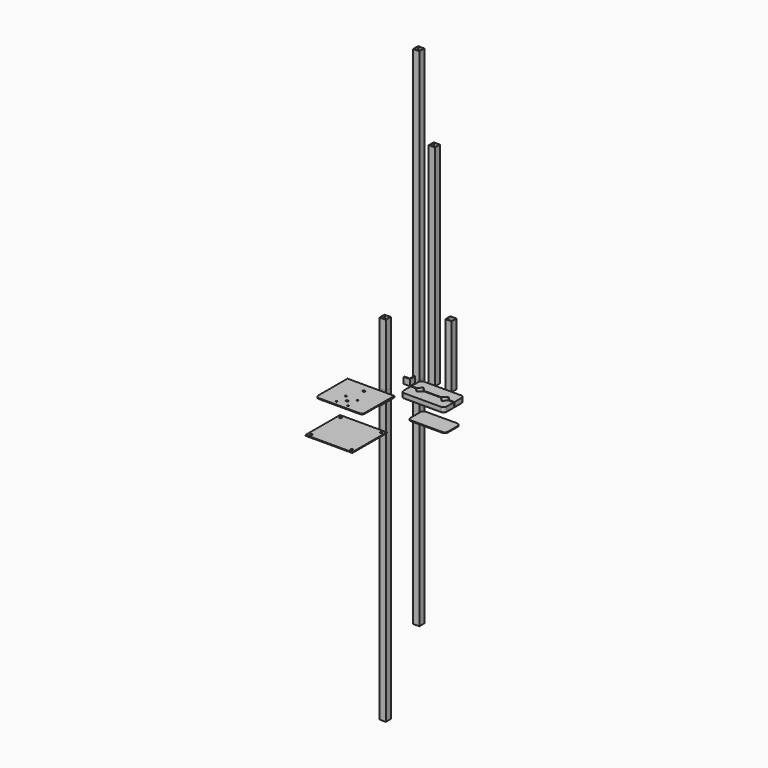
from build123d import *

# Parameters (mm, degrees)
F0_W      = 25.4
F0_H      = 25.4
F1_DEPTH  = 1181.1
F2_DEPTH  = 856.615
F3_DEPTH  = 25.4
F0_R      = 4.7625
F4_DEPTH  = 15.875
F5_DEPTH  = 3.175
F8_DEPTH  = 254
F10_DEPTH = 254
F11_DEPTH = 1187.45
F12_DEPTH = 880.2878
F0_R_2    = 3.175
F13_DEPTH = 3.175
F14_DEPTH = 3.175
F0_W_2    = 190.5
F0_H_2    = 175.514
F15_DEPTH = 3.175
F16_DEPTH = 3.175


# Not quite as in the source:
# - a feature names something its author has since deleted; it is built from what else it names


with BuildPart() as f1:
    # F0 (on Top) → F1 (new body)
    with BuildSketch(Plane.XY):
        with Locations((-44.022594732, 33.2031734467)):
            Rectangle(F0_W, F0_H)
        with BuildLine():
            ThreePointArc((-55.135094732, 42.7281734467), (-54.6701267472, 43.8507054618), (-53.547594732, 44.3156734467))
            Line((-53.547594732, 44.3156734467), (-34.497594732, 44.3156734467))
            ThreePointArc((-34.497594732, 44.3156734467), (-33.3750627169, 43.8507054618), (-32.910094732, 42.7281734467))
            Line((-32.910094732, 42.7281734467), (-32.910094732, 23.6781734467))
            ThreePointArc((-32.910094732, 23.6781734467), (-33.3750627169, 22.5556414315), (-34.497594732, 22.0906734467))
            Line((-34.497594732, 22.0906734467), (-53.547594732, 22.0906734467))
            ThreePointArc((-53.547594732, 22.0906734467), (-54.6701267472, 22.5556414315), (-55.135094732, 23.6781734467))
            Line((-55.135094732, 23.6781734467), (-55.135094732, 42.7281734467))
        make_face(mode=Mode.SUBTRACT)
    extrude(amount=F1_DEPTH)


with BuildPart() as f2:
    # F0 (on Top) → F2 (new body)
    with BuildSketch(Plane.XY):
        with Locations((19.2820195436, 33.6916345775)):
            Rectangle(F0_W, F0_H)
        with BuildLine():
            ThreePointArc((28.8070195436, 44.8041345775), (29.9295515588, 44.3391665926), (30.3945195436, 43.2166345775))
            Line((30.3945195436, 43.2166345775), (30.3945195436, 24.1666345775))
            ThreePointArc((30.3945195436, 24.1666345775), (29.9295515588, 23.0441025624), (28.8070195436, 22.5791345775))
            Line((28.8070195436, 22.5791345775), (9.7570195436, 22.5791345775))
            ThreePointArc((9.7570195436, 22.5791345775), (8.6344875285, 23.0441025624), (8.1695195436, 24.1666345775))
            Line((8.1695195436, 24.1666345775), (8.1695195436, 43.2166345775))
            ThreePointArc((8.1695195436, 43.2166345775), (8.6344875285, 44.3391665926), (9.7570195436, 44.8041345775))
            Line((9.7570195436, 44.8041345775), (28.8070195436, 44.8041345775))
        make_face(mode=Mode.SUBTRACT)
    extrude(amount=F2_DEPTH)


with BuildPart() as f3:
    # F0 (on Top) → F3 (new body)
    with BuildSketch(Plane.XY):
        with BuildLine():
            Line((-30.7852902532, -2.1858640671), (-33.9602902532, -2.1858640671))
            Line((-33.9602902532, -2.1858640671), (-33.9602902532, -21.2358640671))
            ThreePointArc((-33.9602902532, -21.2358640671), (-34.8902262229, -23.4809280973), (-37.1352902532, -24.4108640671))
            Line((-37.1352902532, -24.4108640671), (-56.1852902532, -24.4108640671))
            Line((-56.1852902532, -24.4108640671), (-56.1852902532, -27.5858640671))
            Line((-56.1852902532, -27.5858640671), (-30.7852902532, -27.5858640671))
            Line((-30.7852902532, -27.5858640671), (-30.7852902532, -2.1858640671))
        make_face()
    extrude(amount=F3_DEPTH)


with BuildPart() as f4:
    # F0 (on Top) → F4 (new body)
    with BuildSketch(Plane.XY):
        with BuildLine():
            Line((153.8100352997, 1.1835222483), (3.6851863311, 1.1835222483))
            ThreePointArc((3.6851863311, 1.1835222483), (-5.2950697899, -2.5362216307), (-9.0148136689, -11.5164777517))
            Line((-9.0148136689, -11.5164777517), (-9.0148136689, -48.0289777517))
            Line((-9.0148136689, -48.0289777517), (11.3940863311, -48.0289777517))
            Line((11.3940863311, -48.0289777517), (27.7670985733, -31.6559655096))
            Line((27.7670985733, -31.6559655096), (44.1401108154, -48.0289777517))
            Line((44.1401108154, -48.0289777517), (113.3551108154, -48.0289777517))
            Line((113.3551108154, -48.0289777517), (129.7281230576, -31.6559655096))
            Line((129.7281230576, -31.6559655096), (146.1011352997, -48.0289777517))
            Line((146.1011352997, -48.0289777517), (166.5100352997, -48.0289777517))
            Line((166.5100352997, -48.0289777517), (166.5100352997, -11.5164777517))
            ThreePointArc((166.5100352997, -11.5164777517), (162.7902914208, -2.5362216307), (153.8100352997, 1.1835222483))
        make_face()
        with Locations((3.6851863311, -11.5164777517)):
            Circle(F0_R, mode=Mode.SUBTRACT)
        with Locations((153.8100352997, -11.5164777517)):
            Circle(F0_R, mode=Mode.SUBTRACT)
        with Locations((3.6851863311, -11.5164777517)):
            Circle(F0_R)
        with Locations((153.8100352997, -11.5164777517)):
            Circle(F0_R)
    extrude(amount=F4_DEPTH)


with BuildPart() as f4b:
    # F0 (on Top) → F4, piece 2 (new body)
    with BuildSketch(Plane.XY):
        with BuildLine():
            Line((11.3940863311, -51.2039777517), (-9.0148136689, -51.2039777517))
            Line((-9.0148136689, -51.2039777517), (-9.0148136689, -87.7164777517))
            ThreePointArc((-9.0148136689, -87.7164777517), (-5.2950697899, -96.6967338728), (3.6851863311, -100.4164777517))
            Line((3.6851863311, -100.4164777517), (153.8100352997, -100.4164777517))
            ThreePointArc((153.8100352997, -100.4164777517), (162.7902914208, -96.6967338728), (166.5100352997, -87.7164777517))
            Line((166.5100352997, -87.7164777517), (166.5100352997, -51.2039777517))
            Line((166.5100352997, -51.2039777517), (146.1011352997, -51.2039777517))
            Line((146.1011352997, -51.2039777517), (129.7281230576, -67.5769899939))
            Line((129.7281230576, -67.5769899939), (113.3551108154, -51.2039777517))
            Line((113.3551108154, -51.2039777517), (44.1401108154, -51.2039777517))
            Line((44.1401108154, -51.2039777517), (27.7670985733, -67.5769899939))
            Line((27.7670985733, -67.5769899939), (11.3940863311, -51.2039777517))
        make_face()
        with Locations((3.6851863311, -87.7164777517)):
            Circle(F0_R, mode=Mode.SUBTRACT)
        with Locations((153.8100352997, -87.7164777517)):
            Circle(F0_R, mode=Mode.SUBTRACT)
        with Locations((153.8100352997, -87.7164777517)):
            Circle(F0_R)
        with Locations((3.6851863311, -87.7164777517)):
            Circle(F0_R)
    extrude(amount=F4_DEPTH)


with BuildPart() as f5:
    # F0 (on Top) → F5 (new body)
    with BuildSketch(Plane.XY):
        with BuildLine():
            Line((153.8100352997, 1.1835222483), (3.6851863311, 1.1835222483))
            ThreePointArc((3.6851863311, 1.1835222483), (-5.2950697899, -2.5362216307), (-9.0148136689, -11.5164777517))
            Line((-9.0148136689, -11.5164777517), (-9.0148136689, -48.0289777517))
            Line((-9.0148136689, -48.0289777517), (11.3940863311, -48.0289777517))
            Line((11.3940863311, -48.0289777517), (27.7670985733, -31.6559655096))
            Line((27.7670985733, -31.6559655096), (44.1401108154, -48.0289777517))
            Line((44.1401108154, -48.0289777517), (113.3551108154, -48.0289777517))
            Line((113.3551108154, -48.0289777517), (129.7281230576, -31.6559655096))
            Line((129.7281230576, -31.6559655096), (146.1011352997, -48.0289777517))
            Line((146.1011352997, -48.0289777517), (166.5100352997, -48.0289777517))
            Line((166.5100352997, -48.0289777517), (166.5100352997, -11.5164777517))
            ThreePointArc((166.5100352997, -11.5164777517), (162.7902914208, -2.5362216307), (153.8100352997, 1.1835222483))
        make_face()
        with Locations((3.6851863311, -11.5164777517)):
            Circle(F0_R, mode=Mode.SUBTRACT)
        with Locations((153.8100352997, -11.5164777517)):
            Circle(F0_R, mode=Mode.SUBTRACT)
        with BuildLine():
            Line((11.3940863311, -51.2039777517), (-9.0148136689, -51.2039777517))
            Line((-9.0148136689, -51.2039777517), (-9.0148136689, -87.7164777517))
            ThreePointArc((-9.0148136689, -87.7164777517), (-5.2950697899, -96.6967338728), (3.6851863311, -100.4164777517))
            Line((3.6851863311, -100.4164777517), (153.8100352997, -100.4164777517))
            ThreePointArc((153.8100352997, -100.4164777517), (162.7902914208, -96.6967338728), (166.5100352997, -87.7164777517))
            Line((166.5100352997, -87.7164777517), (166.5100352997, -51.2039777517))
            Line((166.5100352997, -51.2039777517), (146.1011352997, -51.2039777517))
            Line((146.1011352997, -51.2039777517), (129.7281230576, -67.5769899939))
            Line((129.7281230576, -67.5769899939), (113.3551108154, -51.2039777517))
            Line((113.3551108154, -51.2039777517), (44.1401108154, -51.2039777517))
            Line((44.1401108154, -51.2039777517), (27.7670985733, -67.5769899939))
            Line((27.7670985733, -67.5769899939), (11.3940863311, -51.2039777517))
        make_face()
        with Locations((3.6851863311, -87.7164777517)):
            Circle(F0_R, mode=Mode.SUBTRACT)
        with Locations((153.8100352997, -87.7164777517)):
            Circle(F0_R, mode=Mode.SUBTRACT)
        Polygon((113.3551108154, -48.0289777517), (44.1401108154, -48.0289777517), (45.7276108154, -49.6164777517), (44.1401108154, -51.2039777517), (113.3551108154, -51.2039777517), (111.7676108154, -49.6164777517), align=None)
        Polygon((11.3940863311, -48.0289777517), (-9.0148136689, -48.0289777517), (-9.0148136689, -51.2039777517), (11.3940863311, -51.2039777517), (9.8065863311, -49.6164777517), align=None)
        Polygon((166.5100352997, -51.2039777517), (166.5100352997, -48.0289777517), (146.1011352997, -48.0289777517), (147.6886352997, -49.6164777517), (146.1011352997, -51.2039777517), align=None)
        Polygon((27.7670985733, -31.6559655096), (11.3940863311, -48.0289777517), (44.1401108154, -48.0289777517), align=None)
        Polygon((44.1401108154, -48.0289777517), (11.3940863311, -48.0289777517), (9.8065863311, -49.6164777517), (11.3940863311, -51.2039777517), (44.1401108154, -51.2039777517), (45.7276108154, -49.6164777517), align=None)
        Polygon((44.1401108154, -51.2039777517), (11.3940863311, -51.2039777517), (27.7670985733, -67.5769899939), align=None)
        Polygon((129.7281230576, -67.5769899939), (146.1011352997, -51.2039777517), (113.3551108154, -51.2039777517), align=None)
        Polygon((147.6886352997, -49.6164777517), (146.1011352997, -48.0289777517), (113.3551108154, -48.0289777517), (111.7676108154, -49.6164777517), (113.3551108154, -51.2039777517), (146.1011352997, -51.2039777517), align=None)
        Polygon((113.3551108154, -48.0289777517), (146.1011352997, -48.0289777517), (129.7281230576, -31.6559655096), align=None)
    extrude(amount=-F5_DEPTH)


with BuildPart() as f8:
    # F0 (on Top) → F8 (new body)
    with BuildSketch(Plane.XY):
        with Locations((85.7311247587, 35.6169353843)):
            Rectangle(F0_W, F0_H)
        with BuildLine():
            Line((95.2561247587, 24.5044353843), (76.2061247587, 24.5044353843))
            ThreePointArc((76.2061247587, 24.5044353843), (75.0835927436, 24.9694033691), (74.6186247587, 26.0919353843))
            Line((74.6186247587, 26.0919353843), (74.6186247587, 45.1419353843))
            ThreePointArc((74.6186247587, 45.1419353843), (75.0835927436, 46.2644673994), (76.2061247587, 46.7294353843))
            Line((76.2061247587, 46.7294353843), (95.2561247587, 46.7294353843))
            ThreePointArc((95.2561247587, 46.7294353843), (96.3786567739, 46.2644673994), (96.8436247587, 45.1419353843))
            Line((96.8436247587, 45.1419353843), (96.8436247587, 26.0919353843))
            ThreePointArc((96.8436247587, 26.0919353843), (96.3786567739, 24.9694033691), (95.2561247587, 24.5044353843))
        make_face(mode=Mode.SUBTRACT)
    extrude(amount=F8_DEPTH)


with BuildPart() as f10:
    # F0 (on Top) → F10 (new body)
    with BuildSketch(Plane.XY):
        with Locations((-84.5126371503, -86.7445782954)):
            Rectangle(F0_W, F0_H)
        with BuildLine():
            ThreePointArc((-74.9876371503, -75.6320782954), (-73.8651051352, -76.0970462802), (-73.4001371503, -77.2195782954))
            Line((-73.4001371503, -77.2195782954), (-73.4001371503, -96.2695782954))
            ThreePointArc((-73.4001371503, -96.2695782954), (-73.8651051352, -97.3921103105), (-74.9876371503, -97.8570782954))
            Line((-74.9876371503, -97.8570782954), (-94.0376371503, -97.8570782954))
            ThreePointArc((-94.0376371503, -97.8570782954), (-95.1601691654, -97.3921103105), (-95.6251371503, -96.2695782954))
            Line((-95.6251371503, -96.2695782954), (-95.6251371503, -77.2195782954))
            ThreePointArc((-95.6251371503, -77.2195782954), (-95.1601691654, -76.0970462802), (-94.0376371503, -75.6320782954))
            Line((-94.0376371503, -75.6320782954), (-74.9876371503, -75.6320782954))
        make_face(mode=Mode.SUBTRACT)
    extrude(amount=F10_DEPTH)


with BuildPart() as f11:
    # F0 (on Top) → F11 (new body)
    with BuildSketch(Plane.XY):
        with Locations((-84.5126371503, -86.7445782954)):
            Rectangle(F0_W, F0_H)
        with BuildLine():
            ThreePointArc((-74.9876371503, -75.6320782954), (-73.8651051352, -76.0970462802), (-73.4001371503, -77.2195782954))
            Line((-73.4001371503, -77.2195782954), (-73.4001371503, -96.2695782954))
            ThreePointArc((-73.4001371503, -96.2695782954), (-73.8651051352, -97.3921103105), (-74.9876371503, -97.8570782954))
            Line((-74.9876371503, -97.8570782954), (-94.0376371503, -97.8570782954))
            ThreePointArc((-94.0376371503, -97.8570782954), (-95.1601691654, -97.3921103105), (-95.6251371503, -96.2695782954))
            Line((-95.6251371503, -96.2695782954), (-95.6251371503, -77.2195782954))
            ThreePointArc((-95.6251371503, -77.2195782954), (-95.1601691654, -76.0970462802), (-94.0376371503, -75.6320782954))
            Line((-94.0376371503, -75.6320782954), (-74.9876371503, -75.6320782954))
        make_face(mode=Mode.SUBTRACT)
    extrude(amount=-F11_DEPTH)


with BuildPart() as f12:
    # F0 (on Top) → F12 (new body)
    with BuildSketch(Plane.XY):
        with Locations((-44.022594732, 33.2031734467)):
            Rectangle(F0_W, F0_H)
        with BuildLine():
            ThreePointArc((-55.135094732, 42.7281734467), (-54.6701267472, 43.8507054618), (-53.547594732, 44.3156734467))
            Line((-53.547594732, 44.3156734467), (-34.497594732, 44.3156734467))
            ThreePointArc((-34.497594732, 44.3156734467), (-33.3750627169, 43.8507054618), (-32.910094732, 42.7281734467))
            Line((-32.910094732, 42.7281734467), (-32.910094732, 23.6781734467))
            ThreePointArc((-32.910094732, 23.6781734467), (-33.3750627169, 22.5556414315), (-34.497594732, 22.0906734467))
            Line((-34.497594732, 22.0906734467), (-53.547594732, 22.0906734467))
            ThreePointArc((-53.547594732, 22.0906734467), (-54.6701267472, 22.5556414315), (-55.135094732, 23.6781734467))
            Line((-55.135094732, 23.6781734467), (-55.135094732, 42.7281734467))
        make_face(mode=Mode.SUBTRACT)
    extrude(amount=-F12_DEPTH)


with BuildPart() as f13:
    # F0 (on Top) → F13 (new body)
    with BuildSketch(Plane.XY):
        with BuildLine():
            Line((-140.5062990204, -185.1695782954), (-215.0408358783, -185.1695782954))
            Line((-215.0408358783, -185.1695782954), (-215.0408358783, -264.5445782954))
            ThreePointArc((-215.0408358783, -264.5445782954), (-211.3210919994, -273.5248344164), (-202.3408358783, -277.2445782954))
            Line((-202.3408358783, -277.2445782954), (-37.2408358783, -277.2445782954))
            ThreePointArc((-37.2408358783, -277.2445782954), (-28.2605797572, -273.5248344164), (-24.5408358783, -264.5445782954))
            Line((-24.5408358783, -264.5445782954), (-24.5408358783, -185.1695782954))
            Line((-24.5408358783, -185.1695782954), (-100.3453727362, -185.1695782954))
            ThreePointArc((-100.3453727362, -185.1695782954), (-89.4333706631, -197.6441831176), (-85.5008358783, -213.7445782954))
            ThreePointArc((-85.5008358783, -213.7445782954), (-136.5262310561, -244.7370435106), (-140.5062990204, -185.1695782954))
        make_face()
        with Locations((-143.9990081961, -259.5427506132)):
            Circle(F0_R_2, mode=Mode.SUBTRACT)
        with Locations((-96.8526635605, -259.5427506132)):
            Circle(F0_R_2, mode=Mode.SUBTRACT)
        with Locations((-202.3408358783, -199.4570782954)):
            Circle(F0_R_2, mode=Mode.SUBTRACT)
        with Locations((-37.2408358783, -199.4570782954)):
            Circle(F0_R_2, mode=Mode.SUBTRACT)
        with BuildLine():
            Line((-37.2408358783, -115.3195782954), (-202.3408358783, -115.3195782954))
            Line((-202.3408358783, -115.3195782954), (-215.0408358783, -115.3195782954))
            Line((-215.0408358783, -115.3195782954), (-215.0408358783, -124.8445782954))
            Line((-215.0408358783, -124.8445782954), (-215.0408358783, -185.1695782954))
            Line((-215.0408358783, -185.1695782954), (-140.5062990204, -185.1695782954))
            ThreePointArc((-140.5062990204, -185.1695782954), (-120.4258358783, -178.8195782954), (-100.3453727362, -185.1695782954))
            Line((-100.3453727362, -185.1695782954), (-24.5408358783, -185.1695782954))
            Line((-24.5408358783, -185.1695782954), (-24.5408358783, -124.8445782954))
            Line((-24.5408358783, -124.8445782954), (-24.5408358783, -115.3195782954))
            Line((-24.5408358783, -115.3195782954), (-37.2408358783, -115.3195782954))
        make_face()
        with Locations((-202.3408358783, -145.4820782954)):
            Circle(F0_R_2, mode=Mode.SUBTRACT)
        Polygon((-171.4063481204, -168.2050905375), (-189.3668603626, -150.2445782954), (-171.4063481204, -132.2840660532), (-153.4458358783, -150.2445782954), align=None, mode=Mode.SUBTRACT)
        with Locations((-120.4258358783, -150.2445782954)):
            Circle(F0_R, mode=Mode.SUBTRACT)
        Polygon((-69.4453236362, -168.2050905375), (-87.4058358783, -150.2445782954), (-69.4453236362, -132.2840660532), (-51.484811394, -150.2445782954), align=None, mode=Mode.SUBTRACT)
        with Locations((-37.2408358783, -145.4820782954)):
            Circle(F0_R_2, mode=Mode.SUBTRACT)
        with BuildLine():
            Line((-100.3453727362, -185.1695782954), (-140.5062990204, -185.1695782954))
            ThreePointArc((-140.5062990204, -185.1695782954), (-136.5262310561, -244.7370435106), (-85.5008358783, -213.7445782954))
            ThreePointArc((-85.5008358783, -213.7445782954), (-89.4333706631, -197.6441831176), (-100.3453727362, -185.1695782954))
        make_face()
        with Locations((-120.4258358783, -235.9695782954)):
            Circle(F0_R, mode=Mode.SUBTRACT)
        with Locations((-143.9990081961, -212.3964059776)):
            Circle(F0_R_2, mode=Mode.SUBTRACT)
        with Locations((-96.8526635605, -212.3964059776)):
            Circle(F0_R_2, mode=Mode.SUBTRACT)
        Polygon((-171.4063481204, -132.2840660532), (-189.3668603626, -150.2445782954), (-171.4063481204, -168.2050905375), (-153.4458358783, -150.2445782954), align=None)
        Polygon((-69.4453236362, -132.2840660532), (-87.4058358783, -150.2445782954), (-69.4453236362, -168.2050905375), (-51.484811394, -150.2445782954), align=None)
        with BuildLine():
            ThreePointArc((-100.3453727362, -185.1695782954), (-120.4258358783, -178.8195782954), (-140.5062990204, -185.1695782954))
            Line((-140.5062990204, -185.1695782954), (-100.3453727362, -185.1695782954))
        make_face()
        with Locations((-202.3408358783, -145.4820782954)):
            Circle(F0_R_2)
        with Locations((-202.3408358783, -199.4570782954)):
            Circle(F0_R_2)
        with Locations((-37.2408358783, -199.4570782954)):
            Circle(F0_R_2)
        with Locations((-37.2408358783, -145.4820782954)):
            Circle(F0_R_2)
    extrude(amount=F13_DEPTH)


with BuildPart() as f14:
    # F0 (on Top) → F14 (new body)
    with BuildSketch(Plane.XY):
        with BuildLine():
            Line((-37.2408358783, -115.3195782954), (-202.3408358783, -115.3195782954))
            Line((-202.3408358783, -115.3195782954), (-215.0408358783, -115.3195782954))
            Line((-215.0408358783, -115.3195782954), (-215.0408358783, -124.8445782954))
            Line((-215.0408358783, -124.8445782954), (-215.0408358783, -185.1695782954))
            Line((-215.0408358783, -185.1695782954), (-140.5062990204, -185.1695782954))
            ThreePointArc((-140.5062990204, -185.1695782954), (-120.4258358783, -178.8195782954), (-100.3453727362, -185.1695782954))
            Line((-100.3453727362, -185.1695782954), (-24.5408358783, -185.1695782954))
            Line((-24.5408358783, -185.1695782954), (-24.5408358783, -124.8445782954))
            Line((-24.5408358783, -124.8445782954), (-24.5408358783, -115.3195782954))
            Line((-24.5408358783, -115.3195782954), (-37.2408358783, -115.3195782954))
        make_face()
        with Locations((-202.3408358783, -145.4820782954)):
            Circle(F0_R_2, mode=Mode.SUBTRACT)
        Polygon((-171.4063481204, -168.2050905375), (-189.3668603626, -150.2445782954), (-171.4063481204, -132.2840660532), (-153.4458358783, -150.2445782954), align=None, mode=Mode.SUBTRACT)
        with Locations((-120.4258358783, -150.2445782954)):
            Circle(F0_R, mode=Mode.SUBTRACT)
        Polygon((-69.4453236362, -168.2050905375), (-87.4058358783, -150.2445782954), (-69.4453236362, -132.2840660532), (-51.484811394, -150.2445782954), align=None, mode=Mode.SUBTRACT)
        with Locations((-37.2408358783, -145.4820782954)):
            Circle(F0_R_2, mode=Mode.SUBTRACT)
        Polygon((-171.4063481204, -132.2840660532), (-189.3668603626, -150.2445782954), (-171.4063481204, -168.2050905375), (-153.4458358783, -150.2445782954), align=None)
        Polygon((-69.4453236362, -132.2840660532), (-87.4058358783, -150.2445782954), (-69.4453236362, -168.2050905375), (-51.484811394, -150.2445782954), align=None)
        with Locations((-202.3408358783, -145.4820782954)):
            Circle(F0_R_2)
        with Locations((-37.2408358783, -145.4820782954)):
            Circle(F0_R_2)
    extrude(amount=-F14_DEPTH)


with BuildPart() as f15:
    # F0 (on Top) → F15 (new body)
    with BuildSketch(Plane.XY):
        with Locations((18.171196328, -413.6125734582)):
            Rectangle(F0_W_2, F0_H_2)
        with Locations((-64.378803672, -488.6695734582)):
            Circle(F0_R, mode=Mode.SUBTRACT)
        with Locations((-64.378803672, -338.5555734582)):
            Circle(F0_R, mode=Mode.SUBTRACT)
        with Locations((100.721196328, -488.6695734582)):
            Circle(F0_R, mode=Mode.SUBTRACT)
        with Locations((100.721196328, -338.5555734582)):
            Circle(F0_R, mode=Mode.SUBTRACT)
    extrude(amount=F15_DEPTH)


with BuildPart() as f16:
    # F0 (on Top) → F16 (new body)
    with BuildSketch(Plane.XY):
        with BuildLine():
            Line((249.7534018952, -137.7315354975), (122.7534018952, -137.7315354975))
            ThreePointArc((122.7534018952, -137.7315354975), (113.7731457742, -141.4512793764), (110.0534018952, -150.4315354975))
            Line((110.0534018952, -150.4315354975), (110.0534018952, -201.2315354975))
            ThreePointArc((110.0534018952, -201.2315354975), (113.7731457742, -210.2117916186), (122.7534018952, -213.9315354975))
            Line((122.7534018952, -213.9315354975), (249.7534018952, -213.9315354975))
            ThreePointArc((249.7534018952, -213.9315354975), (258.7336580163, -210.2117916186), (262.4534018952, -201.2315354975))
            Line((262.4534018952, -201.2315354975), (262.4534018952, -150.4315354975))
            ThreePointArc((262.4534018952, -150.4315354975), (258.7336580163, -141.4512793764), (249.7534018952, -137.7315354975))
        make_face()
        Polygon((135.2728896531, -193.7920477396), (117.312377411, -175.8315354975), (135.2728896531, -157.8710232554), (153.2334018952, -175.8315354975), align=None, mode=Mode.SUBTRACT)
        Polygon((237.2339141374, -193.7920477396), (219.2734018952, -175.8315354975), (237.2339141374, -157.8710232554), (255.1944263795, -175.8315354975), align=None, mode=Mode.SUBTRACT)
        Polygon((135.2728896531, -157.8710232554), (117.312377411, -175.8315354975), (135.2728896531, -193.7920477396), (153.2334018952, -175.8315354975), align=None)
        Polygon((237.2339141374, -157.8710232554), (219.2734018952, -175.8315354975), (237.2339141374, -193.7920477396), (255.1944263795, -175.8315354975), align=None)
    extrude(amount=F16_DEPTH)


solid = Compound([f1.part, f2.part, f3.part, f4.part, f4b.part, f5.part, f8.part, f10.part, f11.part, f12.part, f13.part, f14.part, f15.part, f16.part])
